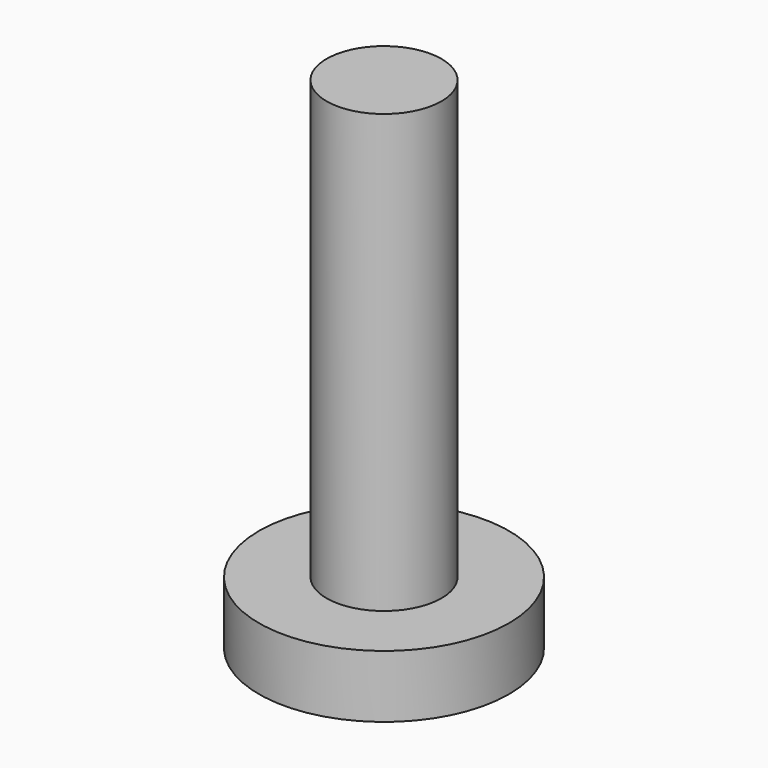
from build123d import *

# Parameters (mm, degrees)
F0_R     = 2.335
F1_DEPTH = 17.78
F2_R     = 5.08
F2_R_2   = 2.335
F3_DEPTH = 2.54


with BuildPart() as f1:
    # F0 (on Top) → F1 (new body)
    with BuildSketch(Plane.XY):
        Circle(F0_R)
    extrude(amount=F1_DEPTH)

    # F2 (on face) → F3 (join)
    with BuildSketch(Plane(origin=(0, 0, 0), x_dir=(1, 0, 0), z_dir=(0, 0, -1))):
        Circle(F2_R)
        Circle(F2_R_2, mode=Mode.SUBTRACT)
        Circle(F2_R_2)
    extrude(amount=F3_DEPTH)


solid = f1.part
